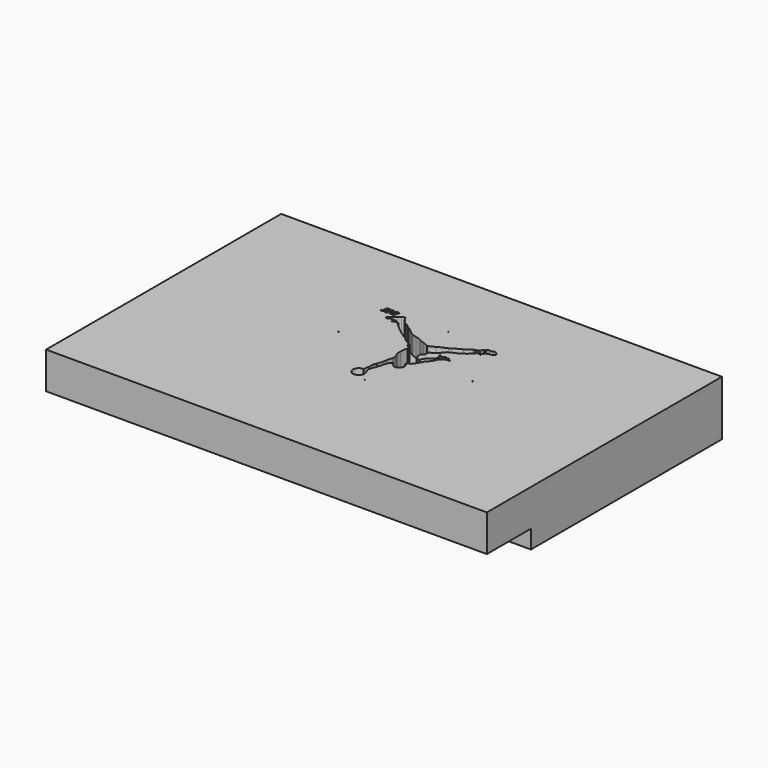
from build123d import *

# Parameters (mm, degrees)
F0_W     = 152.4
F0_H     = 101.6
F1_DEPTH = 19.05
F2_W     = 152.4
F2_H     = 19.05
F3_DEPTH = 6.35
F4_R     = 0.0965371622
F5_DEPTH = 6.35


# Not quite as in the source:
# - ends of sketch curves that miss each other by under 0.0002 mm in the source are joined


with BuildPart() as f1:
    # F0 (on Top) → F1 (new body)
    with BuildSketch(Plane.XY):
        with Locations((-2.0948741585, -7.172193503)):
            Rectangle(F0_W, F0_H)
    extrude(amount=F1_DEPTH)

    # F2 (on face) → F3 (cut)
    with BuildSketch(Plane(origin=(0, 0, 0), x_dir=(1, 0, 0), z_dir=(0, 0, -1))):
        with Locations((-2.0948741585, 48.447193503)):
            Rectangle(F2_W, F2_H)
    extrude(amount=-F3_DEPTH, mode=Mode.SUBTRACT)

    # F4 (on face) → F5 (cut)
    with BuildSketch(Plane.XY.offset(19.05)):
        Polygon((-21.2584489946, 16.3431082703), (-20.5591276135, 18.4025677297), (-21.4882445108, 18.4025677297), (-21.6286049108, 17.9914213622), (-21.2336067649, 17.9914213622), (-21.3876306486, 17.5392835135), (-21.7242492973, 17.5392835135), (-21.8571575432, 17.1492538135), (-21.5192970405, 17.1492538135), (-21.6534481703, 16.7554964919), (-22.0124253405, 16.7554964919), (-22.1527857405, 16.3431082703), align=None)
        Polygon((-18.8971510378, 16.3431082703), (-18.4499826649, 16.3431082703), (-18.1357225378, 17.2709822838), (-18.1481431378, 16.3431082703), (-17.7009747649, 16.3431082703), (-17.0016533838, 18.4025677297), (-17.4475799027, 18.4025677297), (-17.7655655919, 17.4672405324), (-17.7283017324, 18.4025677297), (-18.197828627, 18.4025677297), align=None)
        Polygon((-21.1429308243, 16.3431082703), (-20.6435922243, 16.3431082703), (-20.1243798405, 17.1430424838), (-20.3951658081, 16.3431082703), (-19.8610470568, 16.3431082703), (-19.1617256757, 18.4025677297), (-19.6958433973, 18.4025677297), (-19.9964400405, 17.5206515838), (-19.9219123216, 18.4025677297), (-20.4734201189, 18.4025677297), (-20.5181371622, 17.2734670216), align=None)
        with Locations((23.1689189189, 18.0202702703)):
            Circle(F4_R)
        with Locations((-23.1689189189, 18.0202702703)):
            Circle(F4_R)
        with Locations((-23.1689189189, -18.0202702703)):
            Circle(F4_R)
        with Locations((23.1689189189, -18.0202702703)):
            Circle(F4_R)
        with Locations((23.1689189189, -0.4803699486)):
            Circle(F4_R)
        with Locations((-0.0003624649, 18.0202702703)):
            Circle(F4_R)
        with Locations((-23.1689189189, -0.4803699486)):
            Circle(F4_R)
        with Locations((-0.0003624649, -18.0202702703)):
            Circle(F4_R)
        with BuildLine():
            ThreePointArc((-3.9419806752, -10.3450448162), (-3.9338553566, -10.4511465458), (-3.8919522887, -10.5489613234))
            Line((-3.8919522887, -10.5489613234), (-3.9997791892, -11.5840980243))
            ThreePointArc((-3.9997791892, -11.5840980243), (-4.0620489883, -12.0638953081), (-4.1722996268, -12.5349873691))
            ThreePointArc((-4.1722996268, -12.5349873691), (-4.2317103419, -12.7557842198), (-4.1857767593, -12.9797728957))
            ThreePointArc((-4.1857767593, -12.9797728957), (-4.1347186475, -13.1683923135), (-4.2809406774, -13.2980195258))
            ThreePointArc((-4.2809406774, -13.2980195258), (-5.566970039, -16.8929400959), (-2.4402232824, -14.7018723954))
            ThreePointArc((-2.4402232824, -14.7018723954), (-2.6190032704, -13.9852458307), (-2.9659920907, -13.3332376607))
            ThreePointArc((-2.9659920907, -13.3332376607), (-3.0179767933, -13.0074824834), (-3.117622424, -12.6930157523))
            Line((-3.117622424, -12.6930157523), (-2.6795709405, -10.9175889811))
            ThreePointArc((-2.6795709405, -10.9175889811), (-2.5552563613, -10.8719178146), (-2.4858885849, -10.7590990403))
            Line((-2.4858885849, -10.7590990403), (-2.0787349703, -9.4134215757))
            ThreePointArc((-2.0787349703, -9.4134215757), (-2.0844966147, -9.3526116913), (-2.1201394949, -9.3030066609))
            ThreePointArc((-2.1201394949, -9.3030066609), (-1.9227775345, -8.9652319075), (-1.7526691225, -8.6129425783))
            ThreePointArc((-1.7526691225, -8.6129425783), (-1.7018165564, -8.2609096402), (-1.7181646317, -7.9055986047))
            ThreePointArc((-1.7181646317, -7.9055986047), (-1.3732262139, -7.0781567493), (-1.1315878143, -6.2148760525))
            ThreePointArc((-1.1315878143, -6.2148760525), (-1.1044128192, -6.1550497753), (-1.0798309762, -6.0941122115))
            ThreePointArc((-1.0798309762, -6.0941122115), (-0.6901250043, -5.7928178001), (-0.4242443481, -5.3781420966))
            ThreePointArc((-0.4242443481, -5.3781420966), (-0.353558695, -5.577826024), (-0.2085875429, -5.7322711135))
            ThreePointArc((-0.2085875429, -5.7322711135), (-0.2312257116, -5.8687978131), (-0.2174006404, -6.0064969171))
            ThreePointArc((-0.2174006404, -6.0064969171), (-0.1745992839, -6.0758414621), (-0.106985814, -6.1213282226))
            ThreePointArc((-0.106985814, -6.1213282226), (0.0762855361, -6.1867218616), (0.2661952947, -6.229136679))
            ThreePointArc((0.2661952947, -6.229136679), (0.3545035886, -6.3510127508), (0.4870240633, -6.4223615066))
            ThreePointArc((0.4870240633, -6.4223615066), (0.7054438944, -6.6235174172), (0.9066000997, -6.8419369896))
            ThreePointArc((0.9066000997, -6.8419369896), (1.4603734517, -7.0736101489), (2.0604315783, -7.0572415972))
            ThreePointArc((2.0604315783, -7.0572415972), (2.8583488432, -6.5852535639), (3.3743649716, -5.8150771199))
            ThreePointArc((3.3743649716, -5.8150771199), (3.4588872821, -5.396461525), (3.4295722668, -4.9704055756))
            ThreePointArc((3.4295722668, -4.9704055756), (3.1376684688, -4.3905611726), (2.6566710447, -3.9545921614))
            ThreePointArc((2.6566710447, -3.9545921614), (2.7568759273, -3.7690286411), (2.8167722343, -3.5668221357))
            ThreePointArc((2.8167722343, -3.5668221357), (3.0419010055, -3.2628838305), (3.3502954372, -3.0438990906))
            ThreePointArc((3.3502954372, -3.0438990906), (3.6100031414, -3.010965582), (3.8449527946, -2.8955047749))
            ThreePointArc((3.8449527946, -2.8955047749), (4.0679749644, -2.6910336891), (4.2512805471, -2.4503130495))
            ThreePointArc((4.2512805471, -2.4503130495), (4.7194856727, -1.756348313), (5.1098635587, -1.0158024882))
            ThreePointArc((5.1098635587, -1.0158024882), (5.5640412729, -0.4365158559), (5.8608994576, 0.2370756632))
            ThreePointArc((5.8608994576, 0.2370756632), (7.0626799891, 1.7178141443), (7.9568454926, 3.4022520401))
            ThreePointArc((7.9568454926, 3.4022520401), (8.287589262, 3.8032795043), (8.6724960635, 4.1526517851))
            ThreePointArc((8.6724960635, 4.1526517851), (8.7825092799, 4.2678419248), (8.8809606361, 4.3930577243))
            ThreePointArc((8.8809606361, 4.3930577243), (9.2746379118, 4.6434979771), (9.7077451328, 4.8170498402))
            ThreePointArc((9.7077451328, 4.8170498402), (10.306400854, 4.9141070932), (10.9110409132, 4.9612156407))
            ThreePointArc((10.9110409132, 4.9612156407), (10.9606072989, 5.0160118084), (10.9746333703, 5.0885566638))
            ThreePointArc((10.9746333703, 5.0885566638), (10.9358941446, 5.1806961729), (10.8446089395, 5.2214071421))
            ThreePointArc((10.8446089395, 5.2214071421), (10.1133973805, 5.2845598243), (9.3832503789, 5.2101014439))
            ThreePointArc((9.3832503789, 5.2101014439), (9.3319230539, 5.2286492905), (9.3329410551, 5.2832157401))
            ThreePointArc((9.3329410551, 5.2832157401), (9.5257653342, 5.4030720591), (9.7377110188, 5.4844711882))
            ThreePointArc((9.7377110188, 5.4844711882), (9.8752282145, 5.5403177269), (9.9887145246, 5.6359769788))
            ThreePointArc((9.9887145246, 5.6359769788), (9.9866060059, 5.7313004825), (9.9095699913, 5.787483232))
            ThreePointArc((9.9095699913, 5.787483232), (9.7286220194, 5.8162753028), (9.5455019372, 5.8100964301))
            ThreePointArc((9.5455019372, 5.8100964301), (9.3242057888, 5.7647800594), (9.1189667998, 5.6704268645))
            ThreePointArc((9.1189667998, 5.6704268645), (8.9347967547, 5.5929649469), (8.7390700442, 5.5528398282))
            ThreePointArc((8.7390700442, 5.5528398282), (8.6850508879, 5.5740024204), (8.6870602353, 5.6319844369))
            ThreePointArc((8.6870602353, 5.6319844369), (8.7719706703, 5.7490405803), (8.8408279531, 5.876204212))
            ThreePointArc((8.8408279531, 5.876204212), (8.8424021743, 6.0045261699), (8.7368087295, 6.077457867))
            ThreePointArc((8.7368087295, 6.077457867), (8.6329981913, 6.0749038019), (8.5355542249, 6.0390169958))
            ThreePointArc((8.5355542249, 6.0390169958), (8.4102800447, 5.958199933), (8.295857431, 5.8626359399))
            Line((8.295857431, 5.8626359399), (7.9340500622, 5.4307286919))
            ThreePointArc((7.9340500622, 5.4307286919), (7.8476613342, 5.3910693112), (7.7576690742, 5.4216839997))
            ThreePointArc((7.7576690742, 5.4216839997), (7.5582964586, 5.6332794836), (7.3054111293, 5.7767058767))
            ThreePointArc((7.3054111293, 5.7767058767), (7.0405386531, 5.8377904109), (6.7785304809, 5.7653993152))
            ThreePointArc((6.7785304809, 5.7653993152), (6.7136203742, 5.6418892369), (6.7423500217, 5.5053511443))
            ThreePointArc((6.7423500217, 5.5053511443), (6.8579505418, 5.4338774603), (6.9869695123, 5.3911447667))
            ThreePointArc((6.9869695123, 5.3911447667), (7.1221678309, 5.3294248909), (7.2249260608, 5.2220531954))
            ThreePointArc((7.2249260608, 5.2220531954), (7.241424045, 5.1473752701), (7.2275626492, 5.0721634709))
            ThreePointArc((7.2275626492, 5.0721634709), (7.1959133911, 4.9503775142), (7.1940101881, 4.8245607926))
            ThreePointArc((7.1940101881, 4.8245607926), (7.2167970592, 4.7229085363), (7.2275622738, 4.6192913442))
            ThreePointArc((7.2275622738, 4.6192913442), (6.9908999696, 3.6696486024), (6.354166685, 2.9264114973))
            ThreePointArc((6.354166685, 2.9264114973), (5.072231252, 1.9442039557), (4.1976319765, 0.586571341))
            ThreePointArc((4.1976319765, 0.586571341), (3.8101717639, 0.4551064166), (3.6045845563, 0.1013512907))
            ThreePointArc((3.6045845563, 0.1013512907), (3.4554821163, 0.0990404074), (3.3134529274, 0.1444812416))
            ThreePointArc((3.3134529274, 0.1444812416), (3.0588515557, 0.5770027083), (2.7527537281, 0.9747472197))
            ThreePointArc((2.7527537281, 0.9747472197), (2.7339102365, 1.3807187669), (2.4723988852, 1.6918134868))
            ThreePointArc((2.4723988852, 1.6918134868), (2.3837910507, 2.2329823767), (2.2452200481, 2.7635609814))
            ThreePointArc((2.2452200481, 2.7635609814), (2.4541321738, 2.9955214955), (2.6294624537, 3.253803285))
            ThreePointArc((2.6294624537, 3.253803285), (2.8982339804, 3.2745185749), (3.1241203182, 3.4216316981))
            ThreePointArc((3.1241203182, 3.4216316981), (3.2825211168, 3.6844384221), (3.3714482871, 3.9781219338))
            ThreePointArc((3.3714482871, 3.9781219338), (3.3953836598, 4.2603780567), (3.3846982992, 4.5434456304))
            ThreePointArc((3.3846982992, 4.5434456304), (3.4217928297, 4.9132916967), (3.5790284519, 5.2500987071))
            ThreePointArc((3.5790284519, 5.2500987071), (3.747447362, 5.3953084836), (3.9533331896, 5.4793434371))
            ThreePointArc((3.9533331896, 5.4793434371), (4.3683989664, 5.634183711), (4.6548116813, 5.9721524484))
            ThreePointArc((4.6548116813, 5.9721524484), (6.0520308478, 7.0919844444), (7.1908968715, 8.4737330107))
            ThreePointArc((7.1908968715, 8.4737330107), (7.8954170547, 8.6444920809), (8.4503144351, 9.1109649007))
            ThreePointArc((8.4503144351, 9.1109649007), (10.9086371068, 10.3298152781), (13.0422395839, 12.0551221619))
            ThreePointArc((13.0422395839, 12.0551221619), (13.4055327306, 12.4522454246), (13.8301579479, 12.7829752007))
            ThreePointArc((13.8301579479, 12.7829752007), (13.8769052259, 12.8722777431), (13.8266238502, 12.9596387758))
            ThreePointArc((13.8266238502, 12.9596387758), (13.7768825335, 12.9944101971), (13.8054250869, 13.0479693253))
            ThreePointArc((13.8054250869, 13.0479693253), (13.9345573875, 13.109027042), (14.0350874267, 13.2105005779))
            ThreePointArc((14.0350874267, 13.2105005779), (14.098932369, 13.1408737145), (14.1764178545, 13.0868360715))
            ThreePointArc((14.1764178545, 13.0868360715), (14.2898942769, 13.0450395926), (14.4096133636, 13.0621036371))
            ThreePointArc((14.4096133636, 13.0621036371), (14.5195713923, 13.1521554157), (14.579209197, 13.2811648847))
            ThreePointArc((14.579209197, 13.2811648847), (14.6226580368, 13.3790552282), (14.6816737589, 13.4684277043))
            ThreePointArc((14.6816737589, 13.4684277043), (14.7792931779, 13.5087052722), (14.8795369309, 13.4754942664))
            ThreePointArc((14.8795369309, 13.4754942664), (14.9389691147, 13.4024410867), (14.9537361805, 13.3094307794))
            ThreePointArc((14.9537361805, 13.3094307794), (14.9823427477, 13.0896762453), (15.0491334714, 12.878372124))
            ThreePointArc((15.0491334714, 12.878372124), (15.1076429577, 12.801247666), (15.1975309134, 12.76530769))
            ThreePointArc((15.1975309134, 12.76530769), (15.2771867255, 12.8160230642), (15.3211954848, 12.8995715147))
            ThreePointArc((15.3211954848, 12.8995715147), (15.3289432469, 13.0544570708), (15.2858636252, 13.2034326985))
            ThreePointArc((15.2858636252, 13.2034326985), (15.2554316597, 13.3073032668), (15.250529625, 13.4154291292))
            ThreePointArc((15.250529625, 13.4154291292), (15.2337305656, 13.6006328477), (15.1621991241, 13.7722893614))
            ThreePointArc((15.1621991241, 13.7722893614), (15.1540420537, 13.8544694888), (15.2363968744, 13.8606202771))
            ThreePointArc((15.2363968744, 13.8606202771), (15.3245835114, 13.8322868325), (15.4165933426, 13.8429548104))
            ThreePointArc((15.4165933426, 13.8429548104), (15.5493631351, 13.9155242536), (15.6391894874, 14.0372837618))
            ThreePointArc((15.6391894874, 14.0372837618), (15.6555446765, 14.1497681996), (15.6533220681, 14.2634135798))
            ThreePointArc((15.6533220681, 14.2634135798), (15.8601315924, 14.337603625), (16.0525812576, 14.4436102625))
            Line((16.0525812576, 14.4436102625), (16.2645779919, 14.4436101162))
            ThreePointArc((16.2645779919, 14.4436101162), (16.5980390376, 14.5983178683), (16.9535671042, 14.6917551844))
            Line((16.9535671042, 14.6917551844), (17.2447087297, 14.6974086324))
            ThreePointArc((17.2447087297, 14.6974086324), (17.5965380099, 14.7220741402), (17.9372286283, 14.8132998799))
            ThreePointArc((17.9372286283, 14.8132998799), (18.2228654135, 15.011476512), (18.4601522775, 15.2655578905))
            ThreePointArc((18.4601522775, 15.2655578905), (18.4928334343, 15.4230856351), (18.4686323691, 15.5821370621))
            ThreePointArc((18.4686323691, 15.5821370621), (18.2668568758, 15.9181113659), (18.0218385561, 16.2239839934))
            ThreePointArc((18.0218385561, 16.2239839934), (17.7550463155, 16.4601688723), (17.4453987785, 16.6364634975))
            ThreePointArc((17.4453987785, 16.6364634975), (17.106882354, 16.6954231653), (16.7641832842, 16.6703831901))
            ThreePointArc((16.7641832842, 16.6703831901), (16.614413119, 16.5668458716), (16.4518466153, 16.484850769))
            ThreePointArc((16.4518466153, 16.484850769), (16.003004297, 16.3726322403), (15.5508627129, 16.4707168193))
            ThreePointArc((15.5508627129, 16.4707168193), (15.4448071624, 16.4724365436), (15.3388674624, 16.4671842599))
            ThreePointArc((15.3388674624, 16.4671842599), (15.1920006143, 16.4580000632), (15.0526724601, 16.4106516093))
            ThreePointArc((15.0526724601, 16.4106516093), (14.8985618395, 16.3016711288), (14.7629450949, 16.170389339))
            ThreePointArc((14.7629450949, 16.170389339), (14.6878186603, 16.0747656259), (14.6507618138, 15.958943919))
            ThreePointArc((14.6507618138, 15.958943919), (14.5387907284, 15.9335165954), (14.4873486289, 15.8308630207))
            ThreePointArc((14.4873486289, 15.8308630207), (14.3964374382, 15.6762616587), (14.266518976, 15.5526191299))
            ThreePointArc((14.266518976, 15.5526191299), (14.1858631037, 15.5542026482), (14.1075221006, 15.5349518668))
            ThreePointArc((14.1075221006, 15.5349518668), (13.9170517881, 15.4262757671), (13.7895281638, 15.2478742094))
            ThreePointArc((13.7895281638, 15.2478742094), (13.6552003232, 15.0270510286), (13.4847852011, 14.8327175072))
            ThreePointArc((13.4847852011, 14.8327175072), (13.4000871714, 14.8218175523), (13.3257884712, 14.7797185437))
            ThreePointArc((13.3257884712, 14.7797185437), (13.2336287796, 14.611808815), (13.0872934394, 14.4882240556))
            ThreePointArc((13.0872934394, 14.4882240556), (12.95552414, 14.4437431077), (12.8443809686, 14.3601434894))
            ThreePointArc((12.8443809686, 14.3601434894), (12.71425106, 14.3616652472), (12.5882195653, 14.3292273418))
            ThreePointArc((12.5882195653, 14.3292273418), (12.3909903674, 14.2048358597), (12.2083928011, 14.0598159893))
            ThreePointArc((12.2083928011, 14.0598159893), (12.1487581165, 14.0326832499), (12.0847285568, 14.0465652571))
            ThreePointArc((12.0847285568, 14.0465652571), (12.0276506173, 14.0799794053), (11.9674141528, 14.1072917979))
            ThreePointArc((11.9674141528, 14.1072917979), (11.859358525, 14.1208746196), (11.7582305734, 14.0804562216))
            ThreePointArc((11.7582305734, 14.0804562216), (10.7342435204, 13.2612136595), (9.6340388646, 12.5475908136))
            ThreePointArc((9.6340388646, 12.5475908136), (7.8142188722, 11.5776361262), (6.0654046218, 10.4848389557))
            ThreePointArc((6.0654046218, 10.4848389557), (4.4448092191, 9.8090238061), (2.8894778718, 8.9941618875))
            ThreePointArc((2.8894778718, 8.9941618875), (1.9527603546, 8.4874950174), (0.9755518401, 8.0641576616))
            ThreePointArc((0.9755518401, 8.0641576616), (0.7696458832, 8.0040500074), (0.5577235723, 8.0372020079))
            ThreePointArc((0.5577235723, 8.0372020079), (-0.3022945466, 8.4529696233), (-1.2079344545, 8.7567959833))
            ThreePointArc((-1.2079344545, 8.7567959833), (-1.857920301, 9.0603927193), (-2.5234206184, 9.3282774683))
            ThreePointArc((-2.5234206184, 9.3282774683), (-2.8105313019, 9.4489977192), (-3.0841201053, 9.5978436597))
            ThreePointArc((-3.0841201053, 9.5978436597), (-4.0252195321, 10.0076291155), (-5.0228485582, 10.2491424391))
            ThreePointArc((-5.0228485582, 10.2491424391), (-5.6046701425, 10.3805361012), (-6.1787521228, 10.5424328499))
            ThreePointArc((-6.1787521228, 10.5424328499), (-6.5290440697, 10.7895980401), (-6.9119743554, 10.982366088))
            ThreePointArc((-6.9119743554, 10.982366088), (-7.300412609, 11.2317336539), (-7.6617430292, 11.518977062))
            ThreePointArc((-7.6617430292, 11.518977062), (-8.5674019035, 12.2029928642), (-9.4228551095, 12.9488449808))
            ThreePointArc((-9.4228551095, 12.9488449808), (-9.7130544352, 13.1088316454), (-10.0339366734, 13.191572329))
            ThreePointArc((-10.0339366734, 13.191572329), (-10.7471318023, 13.7954346266), (-11.5002428034, 14.3487167104))
            ThreePointArc((-11.5002428034, 14.3487167104), (-11.75722075, 14.4267677152), (-12.0255369393, 14.4384280098))
            ThreePointArc((-12.0255369393, 14.4384280098), (-12.2344274553, 14.5934069509), (-12.4119883849, 14.7834744616))
            ThreePointArc((-12.4119883849, 14.7834744616), (-12.6979116189, 15.1424140007), (-13.0537725745, 15.432159922))
            ThreePointArc((-13.0537725745, 15.432159922), (-13.343437089, 15.8731960832), (-13.7231620013, 16.2395665866))
            ThreePointArc((-13.7231620013, 16.2395665866), (-13.7261254958, 16.3130817602), (-13.7438642915, 16.3844859701))
            ThreePointArc((-13.7438642915, 16.3844859701), (-13.9291099975, 16.8307079602), (-14.1855226566, 17.2401986026))
            ThreePointArc((-14.1855226566, 17.2401986026), (-14.3207609696, 17.3043628699), (-14.4686912666, 17.2814917535))
            ThreePointArc((-14.4686912666, 17.2814917535), (-14.8408968851, 17.0512810357), (-15.1585504757, 16.750232546))
            ThreePointArc((-15.1585504757, 16.750232546), (-15.5774660708, 16.4171916629), (-16.0487681009, 16.1636548277))
            ThreePointArc((-16.0487681009, 16.1636548277), (-16.6278142039, 15.8539356308), (-17.1600891931, 15.4693532004))
            ThreePointArc((-17.1600891931, 15.4693532004), (-17.8443657398, 14.8950957079), (-18.4762309812, 14.2636272948))
            ThreePointArc((-18.4762309812, 14.2636272948), (-18.492751602, 14.149016051), (-18.4585648763, 14.0383813506))
            ThreePointArc((-18.4585648763, 14.0383813506), (-18.2989936309, 13.8758296314), (-18.0875723824, 13.7910528428))
            ThreePointArc((-18.0875723824, 13.7910528428), (-17.8769202938, 13.7702628024), (-17.6679998443, 13.8043027953))
            ThreePointArc((-17.6679998443, 13.8043027953), (-17.373748749, 13.944035666), (-17.1070935627, 14.1311293305))
            ThreePointArc((-17.1070935627, 14.1311293305), (-16.9571542481, 14.2205142424), (-16.7935161558, 14.2812927257))
            Line((-16.7935161558, 14.2812927257), (-14.8988093514, 14.2251498649))
            ThreePointArc((-14.8988093514, 14.2251498649), (-15.2101817134, 13.7930389006), (-15.6231281723, 13.4566641741))
            ThreePointArc((-15.6231281723, 13.4566641741), (-15.7713157677, 13.3899069743), (-15.9278730098, 13.3462506213))
            ThreePointArc((-15.9278730098, 13.3462506213), (-15.9780881512, 13.2542753124), (-15.905790237, 13.1784206307))
            ThreePointArc((-15.905790237, 13.1784206307), (-15.8305435057, 13.1800392524), (-15.7556259549, 13.1872542419))
            ThreePointArc((-15.7556259549, 13.1872542419), (-15.3240095674, 13.3076352895), (-14.9827246186, 13.5979954364))
            ThreePointArc((-14.9827246186, 13.5979954364), (-14.8833510486, 13.5854930838), (-14.7839782217, 13.5979958574))
            ThreePointArc((-14.7839782217, 13.5979958574), (-14.7028594935, 13.6940231765), (-14.6028980122, 13.7702420993))
            ThreePointArc((-14.6028980122, 13.7702420993), (-14.4502784205, 13.8166192496), (-14.2959439217, 13.7763151541))
            ThreePointArc((-14.2959439217, 13.7763151541), (-14.1515983356, 13.6738106637), (-14.0199089395, 13.5554860793))
            ThreePointArc((-14.0199089395, 13.5554860793), (-13.883022401, 13.5259386306), (-13.7438718404, 13.5416847784))
            ThreePointArc((-13.7438718404, 13.5416847784), (-13.5982657871, 13.4685085873), (-13.5161415376, 13.3277559195))
            ThreePointArc((-13.5161415376, 13.3277559195), (-13.5554551756, 13.2525255108), (-13.5920513665, 13.1759365888))
            ThreePointArc((-13.5920513665, 13.1759365888), (-13.6250954349, 13.0468450245), (-13.5437445212, 12.9413059558))
            ThreePointArc((-13.5437445212, 12.9413059558), (-13.4889894642, 12.9127983356), (-13.4333307014, 12.8860981059))
            ThreePointArc((-13.4333307014, 12.8860981059), (-13.0826855289, 12.6357184292), (-12.7773198213, 12.3317550736))
            ThreePointArc((-12.7773198213, 12.3317550736), (-10.4532122214, 10.3288072761), (-7.9609264893, 8.5394531764))
            ThreePointArc((-7.9609264893, 8.5394531764), (-7.5950735728, 8.3524002411), (-7.1940543213, 8.2628421141))
            ThreePointArc((-7.1940543213, 8.2628421141), (-5.5078534819, 6.7154200392), (-3.4917133745, 5.6323844158))
            ThreePointArc((-3.4917133745, 5.6323844158), (-3.569249916, 5.509971362), (-3.6407723855, 5.3839507301))
            ThreePointArc((-3.6407723855, 5.3839507301), (-3.6604175612, 5.1067549956), (-3.5579615896, 4.8484407162))
            ThreePointArc((-3.5579615896, 4.8484407162), (-3.1966573125, 4.5013439756), (-2.7684970088, 4.24115994))
            ThreePointArc((-2.7684970088, 4.24115994), (-2.6476218681, 3.8735807647), (-2.4841857911, 3.5228480419))
            ThreePointArc((-2.4841857911, 3.5228480419), (-2.761423376, 2.2102915763), (-2.8675087384, 0.872976029))
            ThreePointArc((-2.8675087384, 0.872976029), (-2.8534898831, 0.1936846937), (-2.8005637883, -0.483686776))
            ThreePointArc((-2.8005637883, -0.483686776), (-2.7112977283, -0.841345752), (-2.5383288946, -1.1668762052))
            ThreePointArc((-2.5383288946, -1.1668762052), (-2.3594654248, -1.4887799396), (-2.2301014659, -1.8335684777))
            ThreePointArc((-2.2301014659, -1.8335684777), (-2.1136356585, -2.2927347331), (-2.042833613, -2.7611202995))
            ThreePointArc((-2.042833613, -2.7611202995), (-2.029712627, -3.0844138159), (-2.0428348298, -3.4077072196))
            ThreePointArc((-2.0428348298, -3.4077072196), (-2.0624456996, -3.5501536125), (-2.1090847006, -3.686169621))
            ThreePointArc((-2.1090847006, -3.686169621), (-2.3077971622, -4.0918660184), (-2.4679315814, -4.514279542))
            ThreePointArc((-2.4679315814, -4.514279542), (-2.5853658798, -4.8495543441), (-2.6501157747, -5.1988500054))
            ThreePointArc((-2.6501157747, -5.1988500054), (-2.6645613298, -5.5298980592), (-2.658413787, -5.8612041))
            ThreePointArc((-2.658413787, -5.8612041), (-2.834691319, -6.3777235271), (-2.872338667, -6.9221943343))
            ThreePointArc((-2.872338667, -6.9221943343), (-3.2103831761, -7.7948967108), (-3.43821469, -8.7026278512))
            ThreePointArc((-3.43821469, -8.7026278512), (-3.6766442905, -8.9662051702), (-3.7901598062, -9.3030078228))
            ThreePointArc((-3.7901598062, -9.3030078228), (-3.8989248741, -9.8192395329), (-3.9419806752, -10.3450448162))
        make_face()
    extrude(amount=-F5_DEPTH, mode=Mode.SUBTRACT)


solid = f1.part
